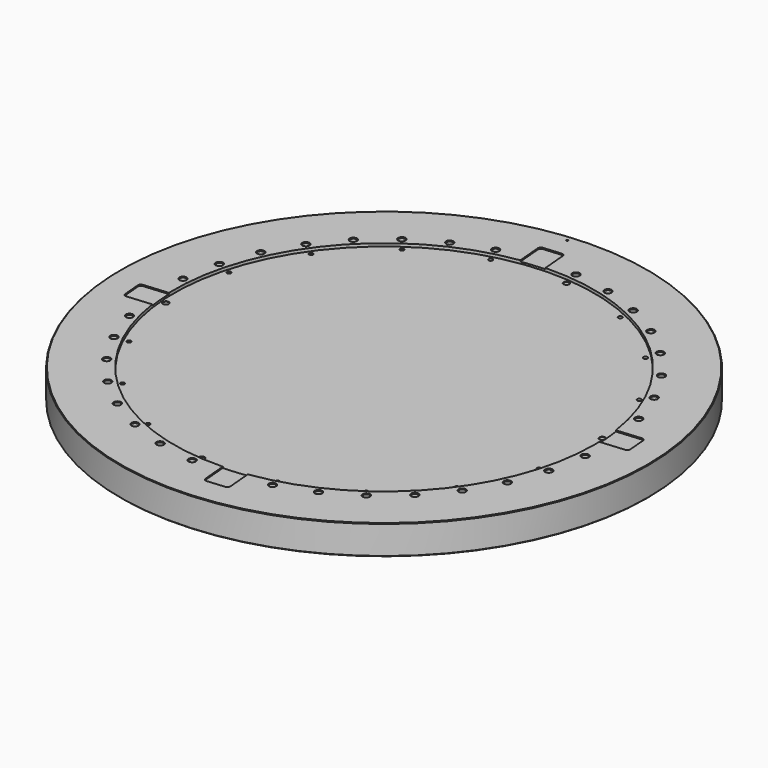
from build123d import *

# Parameters (mm, degrees)
F2_R            = 450
F3_DEPTH        = 50
F4_R            = 358
F5_DEPTH        = 5
F7_D            = 9
F7_DEPTH        = 15
F7_START        = 5
F7_CSINK_D      = 10
F7_CSINK_ANGLE  = 90
F7_TIP          = 2.7038727856
F8_D            = 6.8
F8_DEPTH        = 17.75
F8_START        = 5
F8_TIP          = 2.0429261047
F13_DEPTH       = 2
F14_R           = 1.5
F15_DEPTH       = 60.1
F17_D           = 10.3
F17_DEPTH       = 21.25
F17_CSINK_D     = 12.5
F17_CSINK_ANGLE = 90
F17_TIP         = 3.094432188
F18_SIZE        = 1


with BuildPart() as f3:
    # F2 (on Top) → F3 (new body)
    with BuildSketch(Plane.XY):
        Circle(F2_R)
    extrude(amount=-F3_DEPTH)

    # F4 (on face) → F5 (cut)
    with BuildSketch(Plane.XY):
        Circle(F4_R)
    extrude(amount=-F5_DEPTH, mode=Mode.SUBTRACT)

    # F7
    # its depths count from where the whole tool has entered the part; down to there all is cleared
    with Locations(Plane.XY.offset(-F7_START)):
        with Locations((32.04, 348.53), (348.7987337698, 28.9683589557), (-32.04, -348.53), (-348.7987337698, -28.9683589557)):
            CounterSinkHole(F7_D / 2, F7_CSINK_D / 2, depth=F7_DEPTH, counter_sink_angle=F7_CSINK_ANGLE)
            with Locations((0, 0, -(F7_DEPTH + F7_TIP / 2))):  # 118° drill point
                Cone(0, F7_D / 2, F7_TIP, mode=Mode.SUBTRACT)

    # F8
    # its depths count from where the whole tool has entered the part; down to there all is cleared
    with Locations(Plane.XY.offset(-F8_START)):
        with Locations((149.3120321233, 316.5527437304), (248.5748295616, 246.3945547459), (317.855833981, 146.5175460627), (337.6713585449, -92.0748397688), (285.815833981, -202.0124539373), (199.4867016465, -287.5843847746), (89.0965289833, -338.4693945147), (-149.3120321233, -316.5527437304), (-248.5748295616, -246.3945547459), (-317.855833981, -146.5175460627), (-337.6713585449, 92.0748397688), (-285.815833981, 202.0124539373), (-199.4867016465, 287.5843847746), (-89.0965289833, 338.4693945147)):
            Hole(F8_D / 2, depth=F8_DEPTH)
            with Locations((0, 0, -(F8_DEPTH + F8_TIP / 2))):  # 118° drill point
                Cone(0, F8_D / 2, F8_TIP, mode=Mode.SUBTRACT)

    # F12 (on Top) → F13 (cut)
    with BuildSketch(Plane.XY):
        with BuildLine():
            Line((-11.219122807, 357.8241625204), (-14.8412854475, 399.225670951))
            ThreePointArc((-14.8412854475, 399.225670951), (-16.6083208895, 402.6201144528), (-20.2580376517, 403.7708657277))
            Line((-20.2580376517, 403.7708657277), (-35.2109200701, 402.4626580291))
            Line((-35.2109200701, 402.4626580291), (-31.2017559037, 356.6377019168))
            ThreePointArc((-31.2017559037, 356.6377019168), (-21.2187337001, 357.3706274166), (-11.219122807, 357.8241625204))
        make_face()
        with BuildLine():
            ThreePointArc((-51.0868346246, 354.3361896957), (-41.1603847456, 355.6259590182), (-31.2017559037, 356.6377019168))
            Line((-31.2017559037, 356.6377019168), (-35.2109200701, 402.4626580291))
            Line((-35.2109200701, 402.4626580291), (-50.1638024884, 401.1544503304))
            ThreePointArc((-50.1638024884, 401.1544503304), (-53.5582459903, 399.3874148884), (-54.7089972651, 395.7376981262))
            Line((-54.7089972651, 395.7376981262), (-51.0868346246, 354.3361896957))
        make_face()
        with BuildLine():
            ThreePointArc((-356.6377019168, -31.2017559037), (-357.3706274166, -21.2187337001), (-357.8241625204, -11.219122807))
            Line((-357.8241625204, -11.219122807), (-399.225670951, -14.8412854475))
            ThreePointArc((-399.225670951, -14.8412854475), (-402.6201144528, -16.6083208895), (-403.7708657277, -20.2580376517))
            Line((-403.7708657277, -20.2580376517), (-402.4626580291, -35.2109200701))
            Line((-402.4626580291, -35.2109200701), (-356.6377019168, -31.2017559037))
        make_face()
        with BuildLine():
            ThreePointArc((-354.3361896957, -51.0868346246), (-355.6259590182, -41.1603847456), (-356.6377019168, -31.2017559037))
            Line((-356.6377019168, -31.2017559037), (-402.4626580291, -35.2109200701))
            Line((-402.4626580291, -35.2109200701), (-401.1544503304, -50.1638024884))
            ThreePointArc((-401.1544503304, -50.1638024884), (-399.3874148884, -53.5582459903), (-395.7376981262, -54.7089972651))
            Line((-395.7376981262, -54.7089972651), (-354.3361896957, -51.0868346246))
        make_face()
        with BuildLine():
            ThreePointArc((31.2017559037, -356.6377019168), (21.2187337001, -357.3706274166), (11.219122807, -357.8241625204))
            Line((11.219122807, -357.8241625204), (14.8412854475, -399.225670951))
            ThreePointArc((14.8412854475, -399.225670951), (16.6083208895, -402.6201144528), (20.2580376517, -403.7708657277))
            Line((20.2580376517, -403.7708657277), (35.2109200701, -402.4626580291))
            Line((35.2109200701, -402.4626580291), (31.2017559037, -356.6377019168))
        make_face()
        with BuildLine():
            ThreePointArc((51.0868346246, -354.3361896957), (41.1603847456, -355.6259590182), (31.2017559037, -356.6377019168))
            Line((31.2017559037, -356.6377019168), (35.2109200701, -402.4626580291))
            Line((35.2109200701, -402.4626580291), (50.1638024884, -401.1544503304))
            ThreePointArc((50.1638024884, -401.1544503304), (53.5582459903, -399.3874148884), (54.7089972651, -395.7376981262))
            Line((54.7089972651, -395.7376981262), (51.0868346246, -354.3361896957))
        make_face()
        with BuildLine():
            ThreePointArc((356.6377019168, 31.2017559037), (357.3706274166, 21.2187337001), (357.8241625204, 11.219122807))
            Line((357.8241625204, 11.219122807), (399.225670951, 14.8412854475))
            ThreePointArc((399.225670951, 14.8412854475), (402.6201144528, 16.6083208895), (403.7708657277, 20.2580376517))
            Line((403.7708657277, 20.2580376517), (402.4626580291, 35.2109200701))
            Line((402.4626580291, 35.2109200701), (356.6377019168, 31.2017559037))
        make_face()
        with BuildLine():
            ThreePointArc((354.3361896957, 51.0868346246), (355.6259590182, 41.1603847456), (356.6377019168, 31.2017559037))
            Line((356.6377019168, 31.2017559037), (402.4626580291, 35.2109200701))
            Line((402.4626580291, 35.2109200701), (401.1544503304, 50.1638024884))
            ThreePointArc((401.1544503304, 50.1638024884), (399.3874148884, 53.5582459903), (395.7376981262, 54.7089972651))
            Line((395.7376981262, 54.7089972651), (354.3361896957, 51.0868346246))
        make_face()
    extrude(amount=-F13_DEPTH, mode=Mode.SUBTRACT)

    # F14 (on face) → F15 (cut)
    with BuildSketch(Plane.XY):
        with Locations((-38.3425094187, 438.0995035172)):
            Circle(F14_R)
    extrude(amount=-F15_DEPTH, mode=Mode.SUBTRACT)

    # F17
    with Locations(Plane.XY):
        with Locations((156.3841791406, 335.3669544253), (32.2508053269, 368.6283916924), (95.7724915805, 357.4278045458), (212.2442125518, 303.1161490984), (261.6553129653, 261.6553129653), (303.1161490984, 212.2442125518), (335.3669544253, 156.3841791406), (357.4278045458, 95.7724915805), (368.6283916924, -32.2508053269), (357.4278045458, -95.7724915805), (335.3669544253, -156.3841791406), (303.1161490984, -212.2442125518), (95.7724915805, -357.4278045458), (156.3841791406, -335.3669544253), (212.2442125518, -303.1161490984), (261.6553129653, -261.6553129653), (-32.2508053269, -368.6283916924), (-95.7724915805, -357.4278045458), (-156.3841791406, -335.3669544253), (-212.2442125518, -303.1161490984), (-261.6553129653, -261.6553129653), (-303.1161490984, -212.2442125518), (-335.3669544253, -156.3841791406), (-357.4278045458, -95.7724915805), (-368.6283916924, 32.2508053269), (-357.4278045458, 95.7724915805), (-335.3669544253, 156.3841791406), (-303.1161490984, 212.2442125518), (-261.6553129653, 261.6553129653), (-212.2442125518, 303.1161490984), (-156.3841791406, 335.3669544253), (-95.7724915805, 357.4278045458)):
            CounterSinkHole(F17_D / 2, F17_CSINK_D / 2, depth=F17_DEPTH, counter_sink_angle=F17_CSINK_ANGLE)
            with Locations((0, 0, -(F17_DEPTH + F17_TIP / 2))):  # 118° drill point
                Cone(0, F17_D / 2, F17_TIP, mode=Mode.SUBTRACT)

    # F18
    f18_edges = [f3.edges().sort_by_distance(p)[0] for p in [
        (-450, 0, 0),
        (-450, 0, -50),
    ]]
    chamfer(f18_edges, length=F18_SIZE)


solid = f3.part
